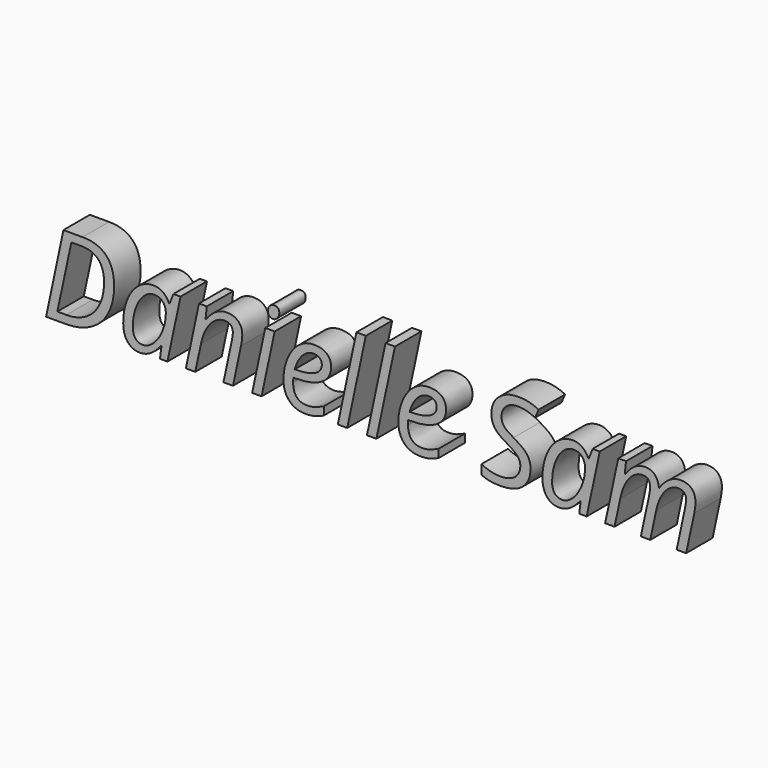
from build123d import *

# Parameters (mm, degrees)
F0_TEXT_SIZE = 34.7222222222
F1_DEPTH     = 10


# Not quite as in the source:
# - Text() gives the source's letters only with a copy of the font that has no kerning and outlines rounded to 1/6400 em; it was checked with that copy


with BuildPart() as f1:
    # F0 (on Front) → F1 (new body)
    with BuildSketch(Plane.XZ):
        with Locations((-13.9025540348, 0)):
            Text('Danielle Sam', F0_TEXT_SIZE, font='Open Sans', font_style=FontStyle.ITALIC, text_align=(TextAlign.LEFT, TextAlign.BOTTOM))
    extrude(amount=-F1_DEPTH)


solid = f1.part
